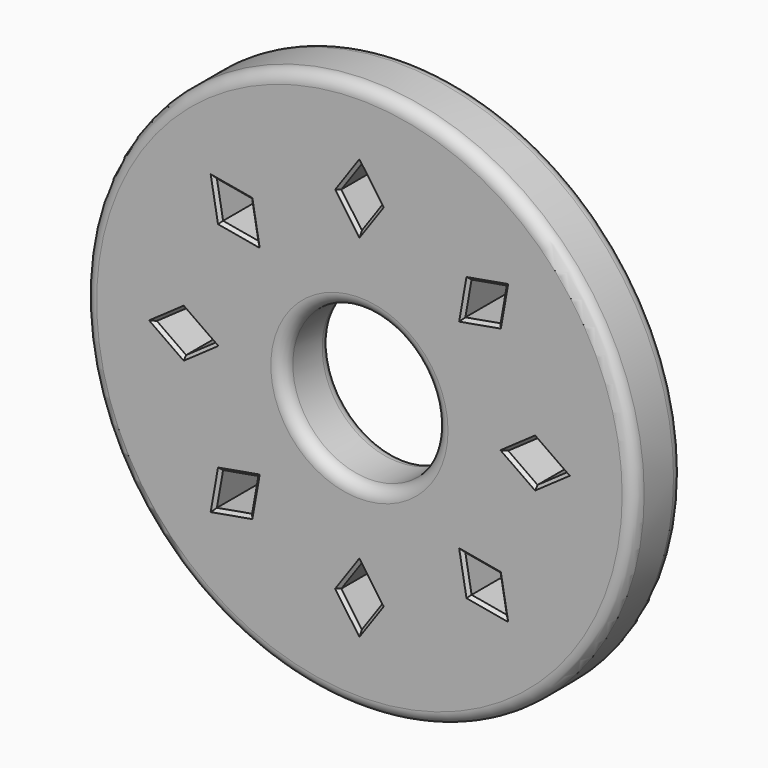
from build123d import *

# Parameters (mm, degrees)
F0_R            = 45
F0_R_2          = 12.5
F1_DEPTH        = 5
F3_DEPTH        = 10.001
F3_COPIES_COUNT = 8
F4_SIZE         = 0.5
F5_R            = 2


# Not quite as in the source:
# - a pattern or mirror of a feature is missing from the dataset's text; its kind, count and spacing are read off the source's solid


with BuildPart() as f1:
    # F0 (on Front) → F1 (new body, symmetric)
    with BuildSketch(Plane.XZ):
        Circle(F0_R)
        Circle(F0_R_2, mode=Mode.SUBTRACT)
    extrude(amount=F1_DEPTH, both=True)

    # F2 (on face) → F3 (cut, through all)
    with BuildSketch(Plane.XZ.offset(5)):
        Polygon((3.36, 28.75), (0, 33.55), (-3.36, 28.75), (0, 23.95), align=None)
    f3 = extrude(amount=-F3_DEPTH, mode=Mode.SUBTRACT)

    # F3_copies: F3 ×8 about axis
    f3_copies_axis = Axis((0, 0, 0), (0, 1, 0))
    for i in range(1, F3_COPIES_COUNT):
        add(f3.rotate(f3_copies_axis, i * 360 / F3_COPIES_COUNT), mode=Mode.SUBTRACT)

    # F4
    f4_edges = [f1.edges().sort_by_distance(p)[0] for p in [
        (1.68, -5, 31.15),
        (-1.68, -5, 31.15),
        (-1.68, -5, 26.35),
        (1.68, -5, 26.35),
        (1.68, 5, 31.15),
        (-1.68, 5, 31.15),
        (-1.68, 5, 26.35),
        (1.68, 5, 26.35),
        (-23.214316, 5, -20.838437),
        (-19.820203, 5, -17.444324),
        (-20.838437, 5, -23.214316),
        (-17.444324, 5, -19.820203),
        (-31.15, 5, 1.68),
        (-26.35, 5, 1.68),
        (-31.15, 5, -1.68),
        (-26.35, 5, -1.68),
        (-1.68, 5, -31.15),
        (-1.68, 5, -26.35),
        (1.68, 5, -31.15),
        (1.68, 5, -26.35),
        (20.838437, 5, -23.214316),
        (17.444324, 5, -19.820203),
        (23.214316, 5, -20.838437),
        (19.820203, 5, -17.444324),
        (-20.838437, 5, 23.214316),
        (-23.214316, 5, 20.838437),
        (-19.820203, 5, 17.444324),
        (-17.444324, 5, 19.820203),
        (31.15, 5, -1.68),
        (26.35, 5, -1.68),
        (31.15, 5, 1.68),
        (26.35, 5, 1.68),
        (23.214316, 5, 20.838437),
        (19.820203, 5, 17.444324),
        (20.838437, 5, 23.214316),
        (17.444324, 5, 19.820203),
        (-23.214316, -5, -20.838437),
        (-19.820203, -5, -17.444324),
        (-20.838437, -5, -23.214316),
        (-17.444324, -5, -19.820203),
        (-31.15, -5, 1.68),
        (-26.35, -5, 1.68),
        (-31.15, -5, -1.68),
        (-26.35, -5, -1.68),
        (-1.68, -5, -31.15),
        (-1.68, -5, -26.35),
        (1.68, -5, -31.15),
        (1.68, -5, -26.35),
        (20.838437, -5, -23.214316),
        (17.444324, -5, -19.820203),
        (23.214316, -5, -20.838437),
        (19.820203, -5, -17.444324),
        (-20.838437, -5, 23.214316),
        (-23.214316, -5, 20.838437),
        (-19.820203, -5, 17.444324),
        (-17.444324, -5, 19.820203),
        (31.15, -5, -1.68),
        (26.35, -5, -1.68),
        (31.15, -5, 1.68),
        (26.35, -5, 1.68),
        (23.214316, -5, 20.838437),
        (19.820203, -5, 17.444324),
        (20.838437, -5, 23.214316),
        (17.444324, -5, 19.820203),
    ]]
    chamfer(f4_edges, length=F4_SIZE)

    # F5
    f5_edges = [f1.edges().sort_by_distance(p)[0] for p in [
        (-45, -5, 0),
        (-45, 5, 0),
        (-12.5, -5, 0),
        (12.5, 0, 0),
        (-12.5, 5, 0),
    ]]
    fillet(f5_edges, radius=F5_R)


solid = f1.part
